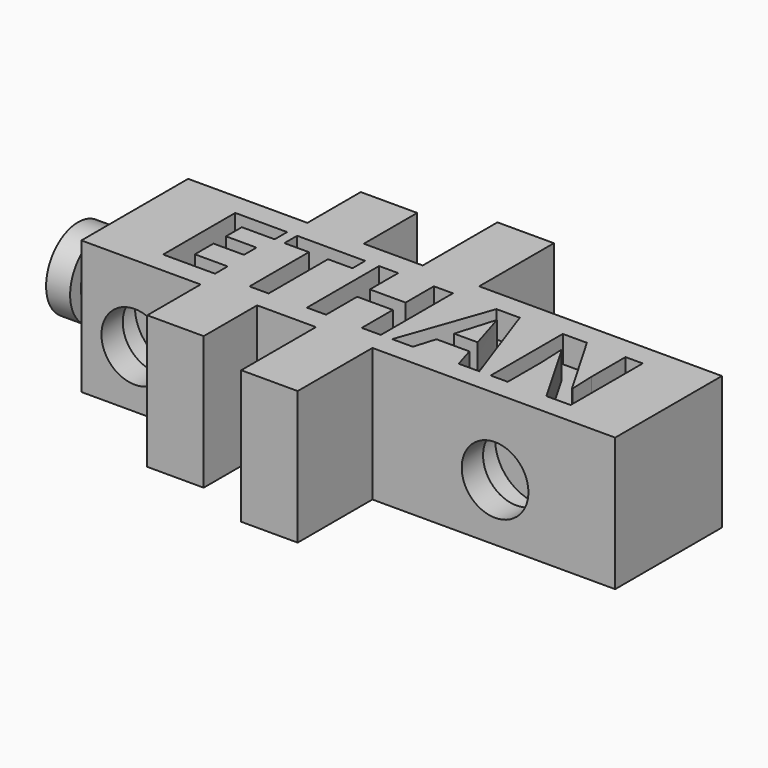
from build123d import *

# Parameters (mm, degrees)
F0_W         = 11.3474776533
F0_H         = 12.7
F0_W_2       = 5.3730774671
F0_H_2       = 6.35
F0_W_3       = 5.6027897402
F0_H_3       = 8.89
F0_W_4       = 23.1035776723
F1_DEPTH     = 12.7
F2_TEXT_SIZE = 12.0158920817
F3_DEPTH     = 2.54
F4_R         = 3.175
F5_DEPTH     = 2.54
F6_R         = 4.0546417353
F7_DEPTH     = 2.54
F8_R         = 3.175
F9_DEPTH     = 2.54
F10_R        = 4.0546417353
F11_DEPTH    = 2.54
F12_R        = 2.54
F13_DEPTH    = 2.794
F14_R        = 3.81
F15_DEPTH    = 2.286
F16_DEPTH    = 2.54


# Not quite as in the source:
# - Text() gives the source's letters only with a copy of the font that has no kerning and outlines rounded to 1/6400 em; it was checked with that copy


with BuildPart() as f1:
    # F0 (on Top) → F1 (new body)
    with BuildSketch(Plane.XY):
        with Locations((-21.4747790945, 0.3907364629)):
            Rectangle(F0_W, F0_H)
        with Locations((-13.1145015343, 9.9157364629)):
            Rectangle(F0_W_2, F0_H_2)
        with Locations((-13.1145015343, 0.3907364629)):
            Rectangle(F0_W_2, F0_H)
        with Locations((-13.1145015343, -9.1342635371)):
            Rectangle(F0_W_2, F0_H_2)
        with Locations((-7.6265679307, 0.3907364629)):
            Rectangle(F0_W_3, F0_H)
        with Locations((-2.138634327, 11.1857364629)):
            Rectangle(F0_W_2, F0_H_3)
        with Locations((-2.138634327, 0.3907364629)):
            Rectangle(F0_W_2, F0_H)
        with Locations((-2.138634327, -10.4042635371)):
            Rectangle(F0_W_2, F0_H_3)
        with Locations((12.0996932427, 0.3907364629)):
            Rectangle(F0_W_4, F0_H)
    extrude(amount=F1_DEPTH)

    # F2 (on face) → F3 (cut)
    with BuildSketch(Plane.XY.offset(12.7)):
        with Locations((-22.0685179212, -3.9349846865)):
            Text('ETHAN', F2_TEXT_SIZE, font='Open Sans', font_style=FontStyle.BOLD, text_align=(TextAlign.LEFT, TextAlign.BOTTOM))
    extrude(amount=-F3_DEPTH, mode=Mode.SUBTRACT)

    # F4 (on face) → F5 (cut)
    with BuildSketch(Plane(origin=(0, 6.7407364629, 0), x_dir=(-1, 0, 0), z_dir=(0, 1, 0))):
        with Locations((22.0685179212, 5.4357722402)):
            Circle(F4_R)
        with Locations((-12.2214820788, 5.4357722402)):
            Circle(F4_R)
    extrude(amount=-F5_DEPTH, mode=Mode.SUBTRACT)

    # F6 (on face) → F7 (cut)
    with BuildSketch(Plane(origin=(0, 4.2007364629, 0), x_dir=(-1, 0, 0), z_dir=(0, 1, 0))):
        with Locations((-12.2214820788, 5.4357722402)):
            Circle(F6_R)
        with Locations((22.0685179212, 5.4357722402)):
            Circle(F6_R)
    extrude(amount=-F7_DEPTH, mode=Mode.SUBTRACT)

    # F8 (on face) → F9 (cut)
    with BuildSketch(Plane.XZ.offset(5.9592635371)):
        with Locations((-22.0685179212, 5.4357722402)):
            Circle(F8_R)
        with Locations((12.2214820788, 5.4357722402)):
            Circle(F8_R)
    extrude(amount=-F9_DEPTH, mode=Mode.SUBTRACT)

    # F10 (on face) → F11 (cut)
    with BuildSketch(Plane.XZ.offset(3.4192635371)):
        with Locations((-22.0685179212, 5.4357722402)):
            Circle(F10_R)
        with Locations((12.2214820788, 5.4357722402)):
            Circle(F10_R)
    extrude(amount=-F11_DEPTH, mode=Mode.SUBTRACT)

    # F12 (on face) → F13 (join)
    with BuildSketch(Plane(origin=(-27.1485179212, 0, 0), x_dir=(0, -1, 0), z_dir=(-1, 0, 0))):
        with Locations((0, 6.35)):
            Circle(F12_R)
    extrude(amount=F13_DEPTH)

    # F14 (on face) → F15 (join)
    with BuildSketch(Plane(origin=(-29.9425179212, 0, 0), x_dir=(0, -1, 0), z_dir=(-1, 0, 0))):
        with Locations((0, 6.35)):
            Circle(F14_R)
    extrude(amount=F15_DEPTH)

    # F2 (on face) → F16 (cut)
    with BuildSketch(Plane.XY.offset(12.7)):
        with Locations((-22.0685179212, -3.9349846865)):
            Text('ETHAN', F2_TEXT_SIZE, font='Open Sans', font_style=FontStyle.BOLD, text_align=(TextAlign.LEFT, TextAlign.BOTTOM))
    extrude(amount=F16_DEPTH, mode=Mode.SUBTRACT)


solid = f1.part
